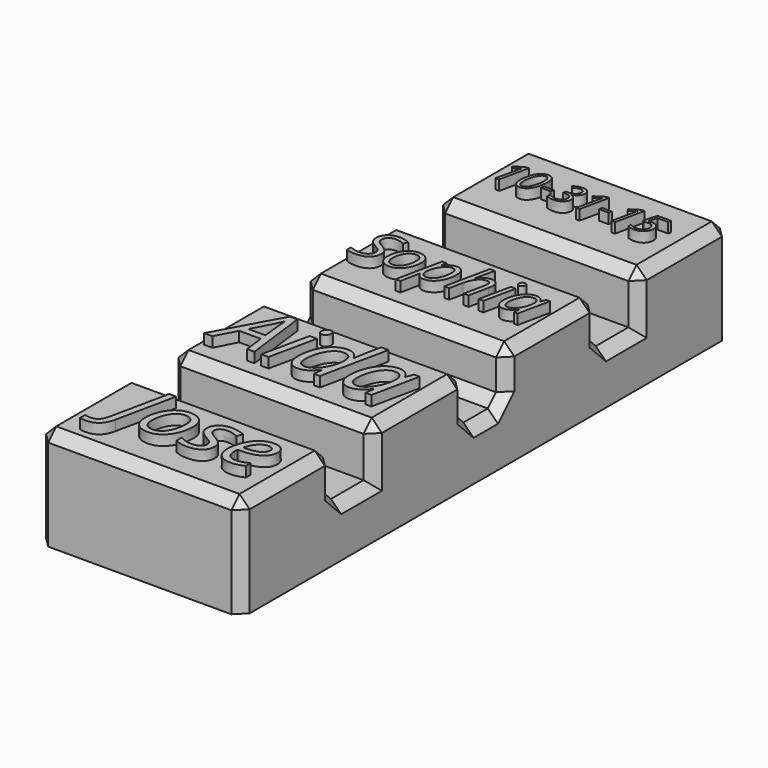
from build123d import *

# Parameters (mm, degrees)
F0_W          = 25.4
F0_H          = 76.2
F1_DEPTH      = 12.7
F2_W          = 6.35
F2_H          = 12.7
F3_DEPTH      = 25.401
F4_SIZE       = 1.27
F5_T          = 2.54
F5_T3_DEPTH   = 6.8760512242
F5_T5_DEPTH   = 7.2797045256
F5_T7_DEPTH   = 6.8760512242
F5_T9_DEPTH   = 7.2797045256
F5_T11_DEPTH  = 6.8760512242
F5_T13_DEPTH  = 6.8760512242
F5_T15_DEPTH  = 6.8760512242
F5_T17_DEPTH  = 27.94
F5_T19_DEPTH  = 7.2797045256
F5_T21_DEPTH  = 6.8760512242
F5_T23_DEPTH  = 6.8760512242
F5_T25_DEPTH  = 6.8760512242
F5_T27_DEPTH  = 7.2797045256
F5_T29_DEPTH  = 6.8760512242
F5_T31_DEPTH  = 6.8760512242
F6_TEXT_SIZE  = 10.4742268041
F7_DEPTH      = 1.27
F8_TEXT_SIZE  = 11.123241846
F9_DEPTH      = 1.27
F10_TEXT_SIZE = 7.4145550375
F11_DEPTH     = 1.27
F12_TEXT_SIZE = 5.1081346479
F13_DEPTH     = 1.27


# Not quite as in the source:
# - a shell that OpenCascade refuses in one call is made with other operations: the cavity is built on its own and cut out
# - Text() gives the source's letters only with a copy of the font that has no kerning and outlines rounded to 1/6400 em; it was checked with that copy


with BuildPart() as f1:
    # F0 (on Top) → F1 (new body)
    with BuildSketch(Plane.XY):
        Rectangle(F0_W, F0_H)
    extrude(amount=F1_DEPTH)

    # F2 (on face) → F3 (cut, through all)
    with BuildSketch(Plane.YZ.offset(12.7)):
        with Locations((0, 12.7)):
            Rectangle(F2_W, F2_H)
        with Locations((20.6502, 12.7)):
            Rectangle(F2_W, F2_H)
        with Locations((-20.6502, 12.7)):
            Rectangle(F2_W, F2_H)
    extrude(amount=-F3_DEPTH, mode=Mode.SUBTRACT)

    # F4
    f4_edges = [f1.edges().sort_by_distance(p)[0] for p in [
        (0, 23.8252, 12.7),
        (-12.7, 30.9626, 12.7),
        (0, 38.1, 12.7),
        (12.7, 30.9626, 12.7),
        (12.7, -20.6502, 6.35),
        (12.7, 0, 6.35),
        (0, 3.175, 6.35),
        (-12.7, 0, 6.35),
        (0, -3.175, 6.35),
        (12.7, 17.4752, 9.525),
        (12.7, 23.8252, 9.525),
        (12.7, -23.8252, 9.525),
        (12.7, -17.4752, 9.525),
        (0, -38.1, 12.7),
        (-12.7, -30.9626, 12.7),
        (0, -23.8252, 12.7),
        (12.7, -30.9626, 12.7),
        (0, -23.8252, 6.35),
        (0, -17.4752, 12.7),
        (-12.7, -10.3251, 12.7),
        (0, -3.175, 12.7),
        (12.7, -10.3251, 12.7),
        (0, 3.175, 12.7),
        (-12.7, 10.3251, 12.7),
        (0, 17.4752, 12.7),
        (12.7, 10.3251, 12.7),
        (0, 17.4752, 6.35),
        (-12.7, 20.6502, 6.35),
        (-12.7, 23.8252, 9.525),
        (-12.7, -23.8252, 9.525),
        (-12.7, -17.4752, 9.525),
        (-12.7, 38.1, 6.35),
        (-12.7, -38.1, 6.35),
        (12.7, -38.1, 6.35),
        (12.7, 38.1, 6.35),
        (-12.7, -20.6502, 6.35),
        (12.7, 20.6502, 6.35),
        (12.7, 3.175, 9.525),
        (12.7, -3.175, 9.525),
        (-12.7, 17.4752, 9.525),
        (-12.7, 3.175, 9.525),
        (-12.7, -3.175, 9.525),
    ]]
    chamfer(f4_edges, length=F4_SIZE)

    # F5: shell of thickness 2.54, made by hand


with BuildPart() as f5_core1:
    # F5_t2: copy of F1
    add(f1.part)

    # the walls: a layer under each face that stays
    f5_faces = [f5_core1.faces().sort_by_distance(p)[0] for p in [
        (12.7, -24.5533333333, 5.715),
        (12.065, -37.465, 5.715),
        (12.065, 37.465, 5.715),
        (12.065, -30.9626, 12.065),
        (12.065, 30.9626, 12.065),
        (12.065, -24.4602, 9.525),
        (12.065, 24.4602, 8.255),
        (12.065, -23.5077, 6.6675),
        (12.065, 21.9202, 5.715),
        (12.065, -19.3802, 5.715),
        (12.065, 17.7927, 6.6675),
        (12.065, -16.8402, 8.255),
        (12.065, 16.8402, 9.525),
        (12.065, -10.3251, 12.065),
        (12.065, 10.3251, 12.065),
        (12.065, -3.81, 9.525),
        (12.065, 3.81, 9.525),
        (12.065, -2.8575, 6.6675),
        (12.065, 2.8575, 6.6675),
        (12.065, 0, 5.715),
        (0, -38.1, 5.715),
        (0, 38.1, 5.715),
        (-12.065, -37.465, 5.715),
        (-12.065, 37.465, 5.715),
        (-12.7, 24.5533333333, 1.905),
        (12.065, -37.1475, 11.7475),
        (12.065, 37.1475, 11.7475),
        (0, -30.9626, 12.7),
        (11.7475, -24.7777, 12.065),
        (12.065, 24.7777, 11.7475),
        (0, 30.9626, 12.7),
        (0, -23.8252, 9.525),
        (0, 23.8252, 8.89),
        (0, -23.1902, 6.985),
        (0, 21.2852, 6.35),
        (0, -20.0152, 6.35),
        (0, 18.1102, 6.985),
        (0, -17.4752, 8.89),
        (11.7475, -16.5227, 12.065),
        (11.7475, 16.5227, 12.065),
        (0, 17.4752, 9.525),
        (0, -10.3251, 12.7),
        (12.065, -4.1275, 11.7475),
        (12.065, 4.1275, 11.7475),
        (0, 10.3251, 12.7),
        (0, -3.175, 9.525),
        (0, 3.175, 9.525),
        (0, -2.54, 6.985),
        (0, 2.54, 6.985),
        (0, 0, 6.35),
        (0, -37.465, 12.065),
        (0, 37.465, 12.065),
        (-12.065, -37.1475, 11.7475),
        (-11.7475, 37.465, 11.7475),
        (-12.065, 30.9626, 12.065),
        (-12.065, -30.9626, 12.065),
        (-12.065, 24.4602, 8.255),
        (-12.065, -24.4602, 9.525),
        (-12.065, 21.9202, 5.715),
        (-12.065, -23.5077, 6.6675),
        (-12.065, 17.7927, 6.6675),
        (-12.065, -19.3802, 5.715),
        (-12.065, 16.8402, 9.525),
        (-12.065, -16.8402, 8.255),
        (-12.065, 10.3251, 12.065),
        (-12.065, -10.3251, 12.065),
        (-12.065, 3.81, 9.525),
        (-12.065, -3.81, 9.525),
        (-12.065, 2.8575, 6.6675),
        (-12.065, -2.8575, 6.6675),
        (-12.065, 0, 5.715),
        (0, -24.4602, 12.065),
        (0, 24.4602, 12.065),
        (0, -16.8402, 12.065),
        (0, 16.8402, 12.065),
        (0, -3.81, 12.065),
        (0, 3.81, 12.065),
        (-12.065, 24.7777, 11.7475),
        (-11.7475, -24.4602, 11.7475),
        (-11.7475, 16.8402, 11.7475),
        (-12.065, -16.5227, 11.7475),
        (-12.065, 4.1275, 11.7475),
        (-11.7475, -3.81, 11.7475),
    ]]
    thicken(f5_faces, amount=-F5_T, mode=Mode.SUBTRACT)

    # F5_s4 → F5_t3 (cut)
    with BuildSketch(Plane(origin=(20.6936512242, -20.6936512242, 0), x_dir=(0, 0, 1), z_dir=(-0.7071067812, 0.7071067812, 0))):
        Polygon((7.6346646968, -8.718590961), (7.62, -11.3047299742), (6.8126933972, -11.3047299742), (6.1535303163, -10.8386312897), align=None)
    extrude(amount=F5_T3_DEPTH, mode=Mode.SUBTRACT)

    # F5_s6 → F5_t5 (cut)
    with BuildSketch(Plane(origin=(12.3715363504, 12.3715363504, -12.3715363504), x_dir=(0.7071067812, -0.7071067812, 0), z_dir=(-0.5773502692, -0.5773502692, 0.5773502692))):
        Polygon((-8.7266299742, 19.5996254641), (-11.3047299742, 19.5776284189), (-11.3047299742, 18.1111587351), (-10.0347299742, 17.3779238932), align=None)
    extrude(amount=F5_T5_DEPTH, mode=Mode.SUBTRACT)

    # F5_s8 → F5_t7 (cut)
    with BuildSketch(Plane(origin=(5.6060512242, 0, -5.6060512242), x_dir=(0, 1, 0), z_dir=(-0.7071067812, 0, 0.7071067812))):
        Polygon((-22.5405353032, -12.6184975827), (-24.0216696837, -10.4984572539), (-23.3625066028, -10.0323585695), (-22.5552, -10.0323585695), align=None)
        Polygon((18.7598646968, -12.6184975827), (18.7452, -10.0323585695), (17.9378933972, -10.0323585695), (17.2787303163, -10.4984572539), align=None)
        Polygon((-1.8903353032, -12.6184975827), (-3.3714696837, -10.4984572539), (-2.7123066028, -10.0323585695), (-1.905, -10.0323585695), align=None)
        Polygon((1.8903353032, -12.6184975827), (3.3714696837, -10.4984572539), (2.7123066028, -10.0323585695), (1.905, -10.0323585695), align=None)
    extrude(amount=F5_T7_DEPTH, mode=Mode.SUBTRACT)

    # F5_s10 → F5_t9 (cut)
    with BuildSketch(Plane(origin=(-1.3952636496, -1.3952636496, 1.3952636496), x_dir=(0.7071067812, -0.7071067812, 0), z_dir=(-0.5773502692, -0.5773502692, 0.5773502692))):
        Polygon((20.4771629316, 2.7388077686), (19.1690629316, 0.5171061978), (17.8990629316, 1.2503410396), (17.8990629316, 2.7168107234), align=None)
    extrude(amount=F5_T9_DEPTH, mode=Mode.SUBTRACT)

    # F5_s12 → F5_t11 (cut)
    with BuildSketch(Plane(origin=(0.0434512242, -0.0434512242, 0), x_dir=(0, 0, 1), z_dir=(-0.7071067812, 0.7071067812, 0))):
        Polygon((7.6346646968, 20.4852019447), (6.1535303163, 18.365161616), (6.8126933972, 17.8990629316), (7.62, 17.8990629316), align=None)
    extrude(amount=F5_T11_DEPTH, mode=Mode.SUBTRACT)

    # F5_s14 → F5_t13 (cut)
    with BuildSketch(Plane(origin=(10.3685512242, -10.3685512242, 0), x_dir=(0, 0, 1), z_dir=(-0.7071067812, 0.7071067812, 0))):
        Polygon((7.6346646968, 5.8833054919), (7.62, 3.2971664787), (6.8126933972, 3.2971664787), (6.1535303163, 3.7632651631), align=None)
    extrude(amount=F5_T13_DEPTH, mode=Mode.SUBTRACT)

    # F5_s16 → F5_t15 (cut)
    with BuildSketch(Plane(origin=(10.3685512242, 10.3685512242, 0), x_dir=(0, 0, 1), z_dir=(-0.7071067812, -0.7071067812, 0))):
        Polygon((7.6346646968, -5.8833054919), (7.62, -3.2971664787), (6.8126933972, -3.2971664787), (6.1535303163, -3.7632651631), align=None)
    extrude(amount=F5_T15_DEPTH, mode=Mode.SUBTRACT)

    # F5_s18 → F5_t17 (cut)
    with BuildSketch(Plane.YZ.offset(-13.97)):
        Polygon((-23.7818394878, 7.6379605122), (-26.3652, 7.62), (-26.3652, 6.5678975516), (-25.6212512242, 5.8239487758), align=None)
        Polygon((23.7998, 6.3754), (26.3652, 6.35), (26.3652, 3.81), (23.8252, 3.81), align=None)
        Polygon((-22.5372394878, 6.3933605122), (-24.3512512242, 4.5539487758), (-23.6073024484, 3.81), (-22.5552, 3.81), align=None)
        Polygon((18.7631605122, 6.3933605122), (18.7452, 3.81), (17.6930975516, 3.81), (16.9491487758, 4.5539487758), align=None)
        Polygon((-17.5006, 6.3754), (-17.4752, 3.81), (-14.9352, 3.81), (-14.9352, 6.35), align=None)
        Polygon((17.5185605122, 7.6379605122), (15.6791487758, 5.8239487758), (14.9352, 6.5678975516), (14.9352, 7.62), align=None)
        Polygon((-3.1316394878, 7.6379605122), (-5.715, 7.62), (-5.715, 6.5678975516), (-4.9710512242, 5.8239487758), align=None)
        Polygon((3.1316394878, 7.6379605122), (5.715, 7.62), (5.715, 6.5678975516), (4.9710512242, 5.8239487758), align=None)
        Polygon((-1.8870394878, 6.3933605122), (-3.7010512242, 4.5539487758), (-2.9571024484, 3.81), (-1.905, 3.81), align=None)
        Polygon((1.8870394878, 6.3933605122), (3.7010512242, 4.5539487758), (2.9571024484, 3.81), (1.905, 3.81), align=None)
    extrude(amount=F5_T17_DEPTH, mode=Mode.SUBTRACT)

    # F5_s20 → F5_t19 (cut)
    with BuildSketch(Plane(origin=(-8.1685969829, 8.1685969829, -8.1685969829), x_dir=(-0.7071067812, -0.7071067812, 0), z_dir=(-0.5773502692, 0.5773502692, -0.5773502692))):
        Polygon((-8.7266299742, 19.5996254641), (-11.3047299742, 19.5776284189), (-11.3047299742, 18.1111587351), (-10.0347299742, 17.3779238932), align=None)
    extrude(amount=F5_T19_DEPTH, mode=Mode.SUBTRACT)

    # F5_s22 → F5_t21 (cut)
    with BuildSketch(Plane(origin=(-20.6936512242, -20.6936512242, 0), x_dir=(0, 0, 1), z_dir=(0.7071067812, 0.7071067812, 0))):
        Polygon((7.6346646968, 8.718590961), (7.62, 11.3047299742), (6.8126933972, 11.3047299742), (6.1535303163, 10.8386312897), align=None)
    extrude(amount=F5_T21_DEPTH, mode=Mode.SUBTRACT)

    # F5_s24 → F5_t23 (cut)
    with BuildSketch(Plane(origin=(-5.6060512242, 0, -5.6060512242), x_dir=(0, 1, 0), z_dir=(0.7071067812, 0, 0.7071067812))):
        Polygon((18.7598646968, 12.6184975827), (18.7452, 10.0323585695), (17.9378933972, 10.0323585695), (17.2787303163, 10.4984572539), align=None)
        Polygon((-22.5405353032, 12.6184975827), (-24.0216696837, 10.4984572539), (-23.3625066028, 10.0323585695), (-22.5552, 10.0323585695), align=None)
        Polygon((1.8903353032, 12.6184975827), (3.3714696837, 10.4984572539), (2.7123066028, 10.0323585695), (1.905, 10.0323585695), align=None)
        Polygon((-1.8903353032, 12.6184975827), (-3.3714696837, 10.4984572539), (-2.7123066028, 10.0323585695), (-1.905, 10.0323585695), align=None)
    extrude(amount=F5_T23_DEPTH, mode=Mode.SUBTRACT)

    # F5_s26 → F5_t25 (cut)
    with BuildSketch(Plane(origin=(-0.0434512242, -0.0434512242, 0), x_dir=(0, 0, 1), z_dir=(0.7071067812, 0.7071067812, 0))):
        Polygon((7.6346646968, -20.4852019447), (6.1535303163, -18.365161616), (6.8126933972, -17.8990629316), (7.62, -17.8990629316), align=None)
    extrude(amount=F5_T25_DEPTH, mode=Mode.SUBTRACT)

    # F5_s28 → F5_t27 (cut)
    with BuildSketch(Plane(origin=(5.5982030171, -5.5982030171, 5.5982030171), x_dir=(-0.7071067812, -0.7071067812, 0), z_dir=(-0.5773502692, 0.5773502692, -0.5773502692))):
        Polygon((20.4771629316, 2.7388077686), (19.1690629316, 0.5171061978), (17.8990629316, 1.2503410396), (17.8990629316, 2.7168107234), align=None)
    extrude(amount=F5_T27_DEPTH, mode=Mode.SUBTRACT)

    # F5_s30 → F5_t29 (cut)
    with BuildSketch(Plane(origin=(-10.3685512242, 10.3685512242, 0), x_dir=(0, 0, 1), z_dir=(0.7071067812, -0.7071067812, 0))):
        Polygon((7.6346646968, 5.8833054919), (7.62, 3.2971664787), (6.8126933972, 3.2971664787), (6.1535303163, 3.7632651631), align=None)
    extrude(amount=F5_T29_DEPTH, mode=Mode.SUBTRACT)

    # F5_s32 → F5_t31 (cut)
    with BuildSketch(Plane(origin=(-10.3685512242, -10.3685512242, 0), x_dir=(0, 0, 1), z_dir=(0.7071067812, 0.7071067812, 0))):
        Polygon((7.6346646968, -5.8833054919), (7.62, -3.2971664787), (6.8126933972, -3.2971664787), (6.1535303163, -3.7632651631), align=None)
    extrude(amount=F5_T31_DEPTH, mode=Mode.SUBTRACT)


with BuildPart() as f1_1:
    add(f1.part)

    # what is left inside the walls is the cavity
    f5_cavity = [f5_core1.part.solids().sort_by_distance(p)[0] for p in [
        (0, -11.853333, 0.0254),
    ]]
    add(f5_cavity, mode=Mode.SUBTRACT)

    # F6 (on face) → F7 (join)
    with BuildSketch(Plane.XY.offset(12.7)):
        with Locations((-7.5922592994, -34.0182356454)):
            Text('Jose', F6_TEXT_SIZE, font='Open Sans', font_style=FontStyle.ITALIC, text_align=(TextAlign.LEFT, TextAlign.BOTTOM))
    extrude(amount=F7_DEPTH)

    # F8 (on face) → F9 (join)
    with BuildSketch(Plane.XY.offset(12.7)):
        with Locations((-10.3016735114, -14.3901878274)):
            Text('Aida', F8_TEXT_SIZE, font='Open Sans', font_style=FontStyle.ITALIC, text_align=(TextAlign.LEFT, TextAlign.BOTTOM))
    extrude(amount=F9_DEPTH)

    # F10 (on face) → F11 (join)
    with BuildSketch(Plane.XY.offset(12.7)):
        with Locations((-11.2057190045, 7.9411830035)):
            Text('Sophia', F10_TEXT_SIZE, font='Open Sans', font_style=FontStyle.ITALIC, text_align=(TextAlign.LEFT, TextAlign.BOTTOM))
    extrude(amount=F11_DEPTH)

    # F12 (on face) → F13 (join)
    with BuildSketch(Plane.XY.offset(12.7)):
        with Locations((-10.2194438058, 28.9055099296)):
            Text('10-31-15', F12_TEXT_SIZE, font='Open Sans', font_style=FontStyle.ITALIC, text_align=(TextAlign.LEFT, TextAlign.BOTTOM))
    extrude(amount=F13_DEPTH)


solid = f1_1.part
